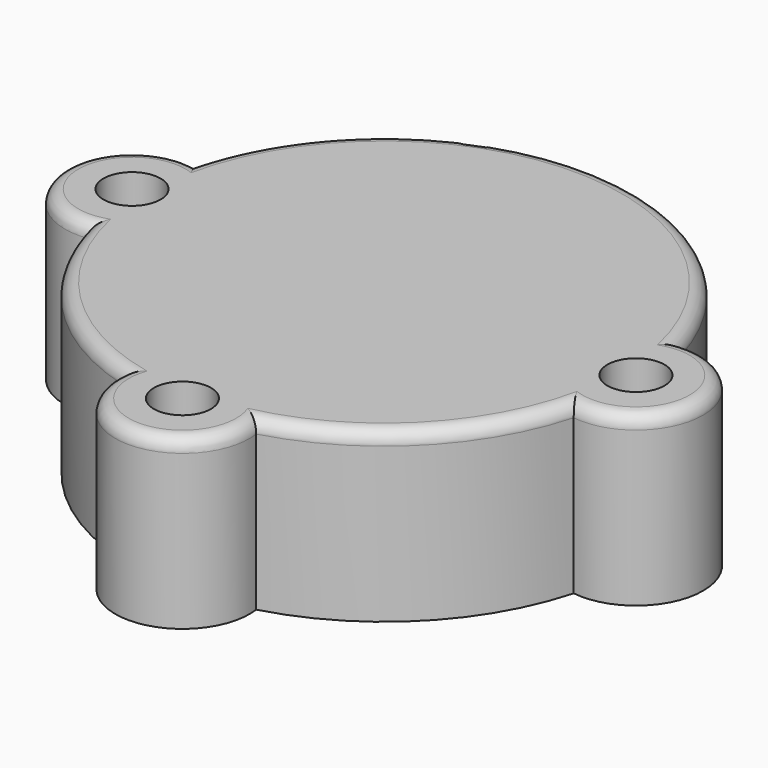
from build123d import *

# Parameters (mm, degrees)
F0_R     = 4.25
F1_DEPTH = 25
F3_R     = 2


# Not quite as in the source:
# - a feature of the source that left no trace in its solid (it failed there, or was rolled back) is left out


with BuildPart() as f1:
    # F0 (on Top) → F1 (new body)
    with BuildSketch(Plane.XY):
        with BuildLine():
            ThreePointArc((36.1666666667, -9.9107124982), (47.5, 0), (36.1666666667, 9.9107124982))
            ThreePointArc((36.1666666667, 9.9107124982), (0, 37.5), (-36.1666666667, 9.9107124982))
            ThreePointArc((-36.1666666667, 9.9107124982), (-47.5, 0), (-36.1666666667, -9.9107124982))
            ThreePointArc((-36.1666666667, -9.9107124982), (-26.5165042945, -26.5165042945), (-9.9107124982, -36.1666666667))
            ThreePointArc((-9.9107124982, -36.1666666667), (0, -47.5), (9.9107124982, -36.1666666667))
            ThreePointArc((9.9107124982, -36.1666666667), (26.5165042945, -26.5165042945), (36.1666666667, -9.9107124982))
        make_face()
        with Locations((0, -37.5)):
            Circle(F0_R, mode=Mode.SUBTRACT)
        with Locations((-37.5, 0)):
            Circle(F0_R, mode=Mode.SUBTRACT)
        with Locations((37.5, 0)):
            Circle(F0_R, mode=Mode.SUBTRACT)
    extrude(amount=F1_DEPTH)

    # F3
    f3_edges = [f1.edges().sort_by_distance(p)[0] for p in [
        (0, -47.5, 25),
        (26.516504, -26.516504, 25),
        (47.5, 0, 25),
        (0, 37.5, 25),
        (-47.5, 0, 25),
        (-26.516504, -26.516504, 25),
    ]]
    fillet(f3_edges, radius=F3_R)


solid = f1.part
